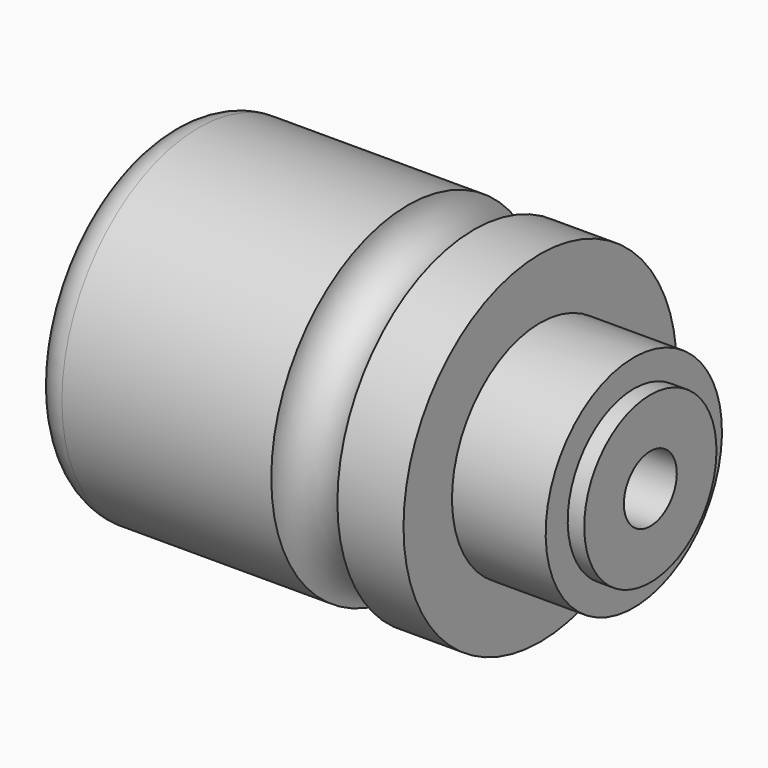
from build123d import *

# Parameters (mm, degrees)
F4_R = 5.99999


# Not quite as in the source:
# - a fillet or chamfer is up to 0.001 mm smaller than in the source, because OpenCascade refuses the exact size


with BuildPart() as f1:
    # F0 (on Front) → F1 (revolve)
    with BuildSketch(Plane.XZ):
        with BuildLine():
            Line((0, 31), (0, 0))
            Line((0, 0), (88, 0))
            Line((88, 0), (88, 15))
            Line((88, 15), (85, 15))
            Line((85, 15), (85, 20))
            Line((85, 20), (68, 20))
            Line((68, 20), (68, 31))
            Line((68, 31), (56, 31))
            ThreePointArc((56, 31), (50, 25), (44, 31))
            Line((44, 31), (0, 31))
        make_face()
    revolve(axis=Axis((44, 0, 0), (-1, 0, 0)))

    # F2 (on Front) → F3 (revolve, cut)
    with BuildSketch(Plane.XZ):
        Polygon((0, 25), (0, 0), (88, 0), (88, 6), (30, 6), (30, 16), (22, 16), (22, 20.5), (15, 20.5), (15, 12.5), (12, 12.5), (12, 16), (1.5, 16), (1.5, 25), align=None)
    revolve(axis=Axis((29.9785251319, 0, 0), (-1, 0, 0)), mode=Mode.SUBTRACT)

    # F4 (radius 6 in the source; OpenCascade refuses exactly that, so slightly less here)
    f4_edges = [f1.edges().sort_by_distance(p)[0] for p in [
        (0, 0, -31),
    ]]
    fillet(f4_edges, radius=F4_R)


solid = f1.part
